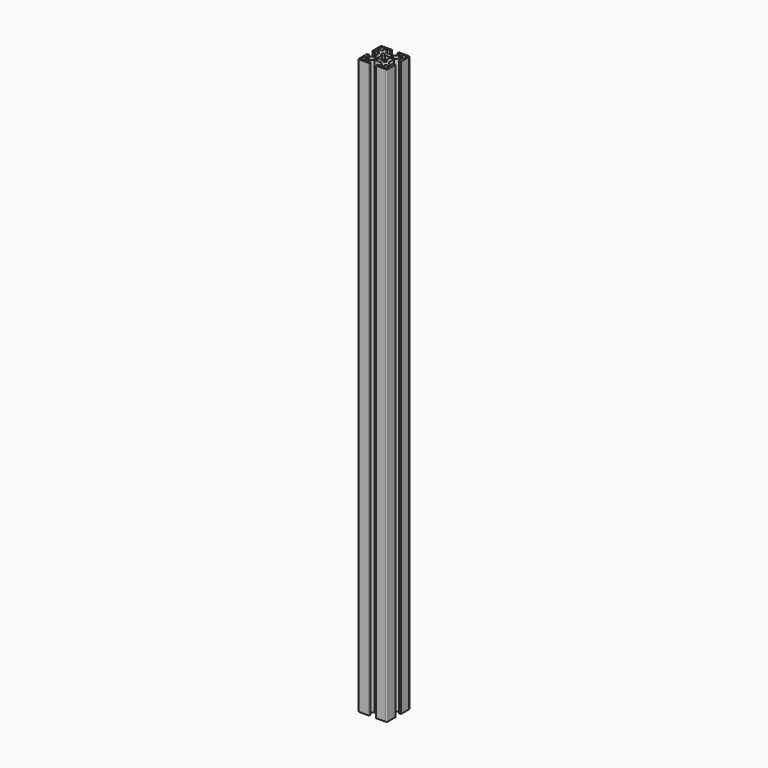
from build123d import *

# Parameters (mm, degrees)
F1_DEPTH = 400


# Not quite as in the source:
# - ends of sketch curves that miss each other by under 0.0002 mm in the source are joined


with BuildPart() as f1:
    # F0 (on Top) → F1 (new body)
    with BuildSketch(Plane.XY):
        with BuildLine():
            ThreePointArc((121.8332443976, 62.5518085142), (121.5989298226, 63.1174939391), (121.0332443976, 63.3518085142))
            Line((121.0332443976, 63.3518085142), (114.4732443976, 63.3518085142))
            ThreePointArc((114.4732443976, 63.3518085142), (114.3035387701, 63.2815141417), (114.2332443976, 63.1118085142))
            Line((114.2332443976, 63.1118085142), (114.2332443976, 61.9918085142))
            ThreePointArc((114.2332443976, 61.9918085142), (114.3035387701, 61.8221028867), (114.4732443976, 61.7518085142))
            Line((114.4732443976, 61.7518085142), (116.6332443976, 61.7518085142))
            Line((116.6332443976, 61.7518085142), (116.6332443976, 61.0003365142))
            Line((116.6332443976, 61.0003365142), (114.1847163976, 58.5518085142))
            Line((114.1847163976, 58.5518085142), (109.4817731976, 58.5518085142))
            Line((109.4817731976, 58.5518085142), (107.0332443976, 61.0003365142))
            Line((107.0332443976, 61.0003365142), (107.0332443976, 61.7518085142))
            Line((107.0332443976, 61.7518085142), (109.1932443976, 61.7518085142))
            ThreePointArc((109.1932443976, 61.7518085142), (109.3629500251, 61.8221028867), (109.4332443976, 61.9918085142))
            Line((109.4332443976, 61.9918085142), (109.4332443976, 63.1118085142))
            ThreePointArc((109.4332443976, 63.1118085142), (109.3629500251, 63.2815141417), (109.1932443976, 63.3518085142))
            Line((109.1932443976, 63.3518085142), (102.6332443976, 63.3518085142))
            ThreePointArc((102.6332443976, 63.3518085142), (102.0675589727, 63.1174939391), (101.8332443976, 62.5518085142))
            Line((101.8332443976, 62.5518085142), (101.8332443976, 55.9918085142))
            ThreePointArc((101.8332443976, 55.9918085142), (101.9035387701, 55.8221028867), (102.0732443976, 55.7518085142))
            Line((102.0732443976, 55.7518085142), (103.1932443976, 55.7518085142))
            ThreePointArc((103.1932443976, 55.7518085142), (103.3629500251, 55.8221028867), (103.4332443976, 55.9918085142))
            Line((103.4332443976, 55.9918085142), (103.4332443976, 58.1518085142))
            Line((103.4332443976, 58.1518085142), (104.1847163976, 58.1518085142))
            Line((104.1847163976, 58.1518085142), (106.6332439976, 55.7032801142))
            Line((106.6332439976, 55.7032801142), (106.6332439976, 51.0003365142))
            Line((106.6332439976, 51.0003365142), (104.1847163976, 48.5518085142))
            Line((104.1847163976, 48.5518085142), (103.4332443976, 48.5518085142))
            Line((103.4332443976, 48.5518085142), (103.4332443976, 50.7118085142))
            ThreePointArc((103.4332443976, 50.7118085142), (103.3629500251, 50.8815141417), (103.1932443976, 50.9518085142))
            Line((103.1932443976, 50.9518085142), (102.0732443976, 50.9518085142))
            ThreePointArc((102.0732443976, 50.9518085142), (101.9035387701, 50.8815141417), (101.8332443976, 50.7118085142))
            Line((101.8332443976, 50.7118085142), (101.8332443976, 44.1518085142))
            ThreePointArc((101.8332443976, 44.1518085142), (102.0675589727, 43.5861230892), (102.6332443976, 43.3518085142))
            Line((102.6332443976, 43.3518085142), (109.1932443976, 43.3518085142))
            ThreePointArc((109.1932443976, 43.3518085142), (109.3629500251, 43.4221028867), (109.4332443976, 43.5918085142))
            Line((109.4332443976, 43.5918085142), (109.4332443976, 44.7118085142))
            ThreePointArc((109.4332443976, 44.7118085142), (109.3629500251, 44.8815141417), (109.1932443976, 44.9518085142))
            Line((109.1932443976, 44.9518085142), (107.0332443976, 44.9518085142))
            Line((107.0332443976, 44.9518085142), (107.0332443976, 45.7032805142))
            Line((107.0332443976, 45.7032805142), (109.4817723976, 48.1518077142))
            Line((109.4817723976, 48.1518077142), (114.1847163976, 48.1518077142))
            Line((114.1847163976, 48.1518077142), (116.6332439976, 45.7032801142))
            Line((116.6332439976, 45.7032801142), (116.6332443976, 44.9518085142))
            Line((116.6332443976, 44.9518085142), (114.4732443976, 44.9518085142))
            ThreePointArc((114.4732443976, 44.9518085142), (114.3035387701, 44.8815141417), (114.2332443976, 44.7118085142))
            Line((114.2332443976, 44.7118085142), (114.2332443976, 43.5918085142))
            ThreePointArc((114.2332443976, 43.5918085142), (114.3035387701, 43.4221028867), (114.4732443976, 43.3518085142))
            Line((114.4732443976, 43.3518085142), (121.0332443976, 43.3518085142))
            ThreePointArc((121.0332443976, 43.3518085142), (121.5989298226, 43.5861230892), (121.8332443976, 44.1518085142))
            Line((121.8332443976, 44.1518085142), (121.8332443976, 50.7118085142))
            ThreePointArc((121.8332443976, 50.7118085142), (121.7629500251, 50.8815141417), (121.5932443976, 50.9518085142))
            Line((121.5932443976, 50.9518085142), (120.4732443976, 50.9518085142))
            ThreePointArc((120.4732443976, 50.9518085142), (120.3035387701, 50.8815141417), (120.2332443976, 50.7118085142))
            Line((120.2332443976, 50.7118085142), (120.2332443976, 48.5518085142))
            Line((120.2332443976, 48.5518085142), (119.4817731976, 48.5518085142))
            Line((119.4817731976, 48.5518085142), (117.0332443976, 51.0003365142))
            Line((117.0332443976, 51.0003365142), (117.0332443976, 55.7032797142))
            Line((117.0332443976, 55.7032797142), (119.4817723976, 58.1518077142))
            Line((119.4817723976, 58.1518077142), (120.2332451976, 58.1518085142))
            Line((120.2332451976, 58.1518085142), (120.2332443976, 55.9918085142))
            ThreePointArc((120.2332443976, 55.9918085142), (120.3035387701, 55.8221028867), (120.4732443976, 55.7518085142))
            Line((120.4732443976, 55.7518085142), (121.5932443976, 55.7518085142))
            ThreePointArc((121.5932443976, 55.7518085142), (121.7629500251, 55.8221028867), (121.8332443976, 55.9918085142))
            Line((121.8332443976, 55.9918085142), (121.8332443976, 62.5518085142))
        make_face()
        with BuildLine():
            Line((105.3844307976, 45.7716237142), (105.8482667976, 45.3077877142))
            ThreePointArc((105.8482667976, 45.3077877142), (105.9696592276, 44.6975055307), (105.4522867976, 44.3518085142))
            Line((105.4522867976, 44.3518085142), (104.0332443976, 44.3518085142))
            ThreePointArc((104.0332443976, 44.3518085142), (103.1847162602, 44.7032803768), (102.8332443976, 45.5518085142))
            Line((102.8332443976, 45.5518085142), (102.8332443976, 46.9708501142))
            ThreePointArc((102.8332443976, 46.9708501142), (103.1789416755, 47.4882226524), (103.7892241951, 47.3668299116))
            Line((103.7892241951, 47.3668299116), (104.2530603976, 46.9029941142))
            Line((104.2530603976, 46.9029941142), (104.8187451976, 47.4686797142))
            ThreePointArc((104.8187451976, 47.4686797142), (105.9501162226, 47.4686795391), (105.9501162226, 46.3373086892))
            Line((105.9501162226, 46.3373086892), (105.3844307976, 45.7716237142))
        make_face(mode=Mode.SUBTRACT)
        with BuildLine():
            ThreePointArc((118.2142027976, 44.3518085142), (117.6968303676, 44.6975055307), (117.8182226001, 45.3077879116))
            Line((117.8182226001, 45.3077879116), (118.2820587976, 45.7716237142))
            Line((118.2820587976, 45.7716237142), (117.7163731976, 46.3373085142))
            ThreePointArc((117.7163731976, 46.3373085142), (117.7163733727, 47.4686795391), (118.8477442226, 47.4686795391))
            Line((118.8477442226, 47.4686795391), (119.4134291976, 46.9029941142))
            Line((119.4134291976, 46.9029941142), (119.8772651976, 47.3668301142))
            ThreePointArc((119.8772651976, 47.3668301142), (120.487547381, 47.4882225442), (120.8332443976, 46.9708501142))
            Line((120.8332443976, 46.9708501142), (120.8332443976, 45.5518085142))
            ThreePointArc((120.8332443976, 45.5518085142), (120.481772535, 44.7032803768), (119.6332443976, 44.3518085142))
            Line((119.6332443976, 44.3518085142), (118.2142027976, 44.3518085142))
        make_face(mode=Mode.SUBTRACT)
        with BuildLine():
            ThreePointArc((110.602965129, 55.7776718494), (111.8332447543, 56.0718085142), (113.0635243025, 55.7776715267))
            ThreePointArc((113.0635243025, 55.7776715267), (113.2098459972, 55.7547084557), (113.3417836251, 55.8220124867))
            Line((113.3417836251, 55.8220124867), (113.7375595976, 56.2177877142))
            ThreePointArc((113.7375595976, 56.2177877142), (115.51020025, 57.0287635666), (114.6992243904, 55.2561228157))
            Line((114.6992243904, 55.2561228157), (114.3034491976, 54.8603469142))
            ThreePointArc((114.3034491976, 54.8603469142), (114.2361451391, 54.7284093138), (114.2591079246, 54.5820874743))
            ThreePointArc((114.2591079246, 54.5820874743), (114.4786884735, 53.9842843173), (114.5532443976, 53.3518085142))
            ThreePointArc((114.5532443976, 53.3518085142), (114.4786883905, 52.7193323641), (114.2591075738, 52.121528932))
            ThreePointArc((114.2591075738, 52.121528932), (114.2361451391, 51.9752069146), (114.3034491701, 51.8432692867))
            Line((114.3034491701, 51.8432692867), (114.6992243976, 51.4474933142))
            ThreePointArc((114.6992243976, 51.4474933142), (115.51020025, 49.6748526618), (113.7375594992, 50.4858285214))
            Line((113.7375594992, 50.4858285214), (113.3417835976, 50.8816037142))
            ThreePointArc((113.3417835976, 50.8816037142), (113.2098461759, 50.9489077442), (113.0635244804, 50.9259451509))
            ThreePointArc((113.0635244804, 50.9259451509), (111.8332447543, 50.6318085142), (110.602965129, 50.9259451789))
            ThreePointArc((110.602965129, 50.9259451789), (110.4566434193, 50.9489077442), (110.3247059701, 50.8816037417))
            Line((110.3247059701, 50.8816037417), (109.9289299976, 50.4858285142))
            ThreePointArc((109.9289299976, 50.4858285142), (108.1562893452, 49.6748526618), (108.9672652048, 51.4474934126))
            Line((108.9672652048, 51.4474934126), (109.3630403976, 51.8432693142))
            ThreePointArc((109.3630403976, 51.8432693142), (109.4303444561, 51.9752069146), (109.4073816706, 52.1215287541))
            ThreePointArc((109.4073816706, 52.1215287541), (109.1132443976, 53.3518081574), (109.4073810624, 54.5820877828))
            ThreePointArc((109.4073810624, 54.5820877828), (109.4303444561, 54.7284093138), (109.3630404251, 54.8603469417))
            Line((109.3630404251, 54.8603469417), (108.9672651976, 55.2561229142))
            ThreePointArc((108.9672651976, 55.2561229142), (108.1562893452, 57.0287635666), (109.928930096, 56.217787707))
            Line((109.928930096, 56.217787707), (110.3247059976, 55.8220125142))
            ThreePointArc((110.3247059976, 55.8220125142), (110.456643598, 55.7547084557), (110.602965129, 55.7776718494))
        make_face(mode=Mode.SUBTRACT)
        with BuildLine():
            ThreePointArc((105.4522867976, 62.3518085142), (105.9696593358, 62.0061112363), (105.8482665951, 61.3958287167))
            Line((105.8482665951, 61.3958287167), (105.3844307976, 60.9319925142))
            Line((105.3844307976, 60.9319925142), (105.9501163976, 60.3663077142))
            ThreePointArc((105.9501163976, 60.3663077142), (105.9501162226, 59.2349366892), (104.8187453727, 59.2349366892))
            Line((104.8187453727, 59.2349366892), (104.2530603976, 59.8006221142))
            Line((104.2530603976, 59.8006221142), (103.7892243976, 59.3367861142))
            ThreePointArc((103.7892243976, 59.3367861142), (103.1789416755, 59.215393576), (102.8332443976, 59.7327661142))
            Line((102.8332443976, 59.7327661142), (102.8332443976, 61.1518085142))
            ThreePointArc((102.8332443976, 61.1518085142), (103.1847162602, 62.0003366516), (104.0332443976, 62.3518085142))
            Line((104.0332443976, 62.3518085142), (105.4522867976, 62.3518085142))
        make_face(mode=Mode.SUBTRACT)
        with BuildLine():
            Line((118.2820587976, 60.9319925142), (117.8182227976, 61.3958285142))
            ThreePointArc((117.8182227976, 61.3958285142), (117.6968302594, 62.0061112363), (118.2142027976, 62.3518085142))
            Line((118.2142027976, 62.3518085142), (119.6332443976, 62.3518085142))
            ThreePointArc((119.6332443976, 62.3518085142), (120.481772535, 62.0003366516), (120.8332443976, 61.1518085142))
            Line((120.8332443976, 61.1518085142), (120.8332443976, 59.7327661142))
            ThreePointArc((120.8332443976, 59.7327661142), (120.487547381, 59.2153936842), (119.8772650001, 59.3367859167))
            Line((119.8772650001, 59.3367859167), (119.4134291976, 59.8006221142))
            Line((119.4134291976, 59.8006221142), (118.8477443976, 59.2349365142))
            ThreePointArc((118.8477443976, 59.2349365142), (117.7163733727, 59.2349366892), (117.7163733727, 60.3663075391))
            Line((117.7163733727, 60.3663075391), (118.2820587976, 60.9319925142))
        make_face(mode=Mode.SUBTRACT)
    extrude(amount=F1_DEPTH)


solid = f1.part
